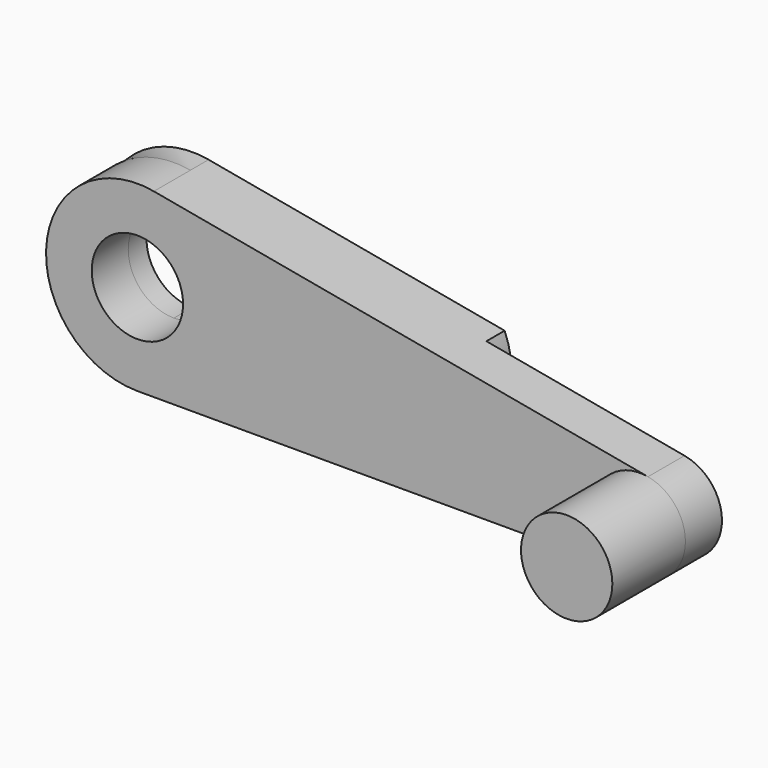
from build123d import *
from build123d import SkipClean  # not in build123d's __all__

# Parameters (mm, degrees)
F0_R     = 2
F1_DEPTH = 1
F2_R     = 2
F3_DEPTH = 4
F5_DEPTH = 1


# Not quite as in the source:
# - after a boolean that leaves OpenCascade's solid faulty, fix() repairs it


with BuildPart() as f1:
    # F0 (on Front) → F1 (new body, symmetric)
    with BuildSketch(Plane.XZ):
        with BuildLine():
            ThreePointArc((0.7213114754, 3.9344262295), (-3.9835728259, 0.3621429842), (0, -4))
            Line((0, -4), (22, -4))
            ThreePointArc((22, -4), (23.9917864129, -2.1810714921), (22.3606557377, -0.0327868852))
            Line((22.3606557377, -0.0327868852), (0.7213114754, 3.9344262295))
        make_face()
        Circle(F0_R, mode=Mode.SUBTRACT)
    extrude(amount=F1_DEPTH, both=True)

    # F2 (on face) → F3 (join)
    with BuildSketch(Plane.XZ.offset(1)):
        with Locations((22, -2)):
            Circle(F2_R)
    with SkipClean():  # cleaning this boolean's faces spoils the solid; the shape is the same uncleaned
        extrude(amount=F3_DEPTH)

    # F4 (on face) → F5 (join)
    with BuildSketch(Plane(origin=(0, 1, 0), x_dir=(-1, 0, 0), z_dir=(0, 1, 0))):
        with BuildLine():
            Line((-0.7213114754, 3.9344262295), (-13.6841453203, 1.5579066913))
            ThreePointArc((-13.6841453203, 1.5579066913), (-13.3340385994, -2.2100195966), (-10, -4))
            Line((-10, -4), (0, -4))
            ThreePointArc((0, -4), (3.9835728259, 0.3621429842), (-0.7213114754, 3.9344262295))
        make_face()
        with BuildLine():
            ThreePointArc((0, 2), (2, 0), (0, -2))
            Line((0, -2), (-10, -2))
            ThreePointArc((-10, -2), (-12, 0), (-10, 2))
            Line((-10, 2), (0, 2))
        make_face(mode=Mode.SUBTRACT)
    extrude(amount=F5_DEPTH)

    add(f1.part.fix(), mode=Mode.REPLACE)


solid = f1.part
